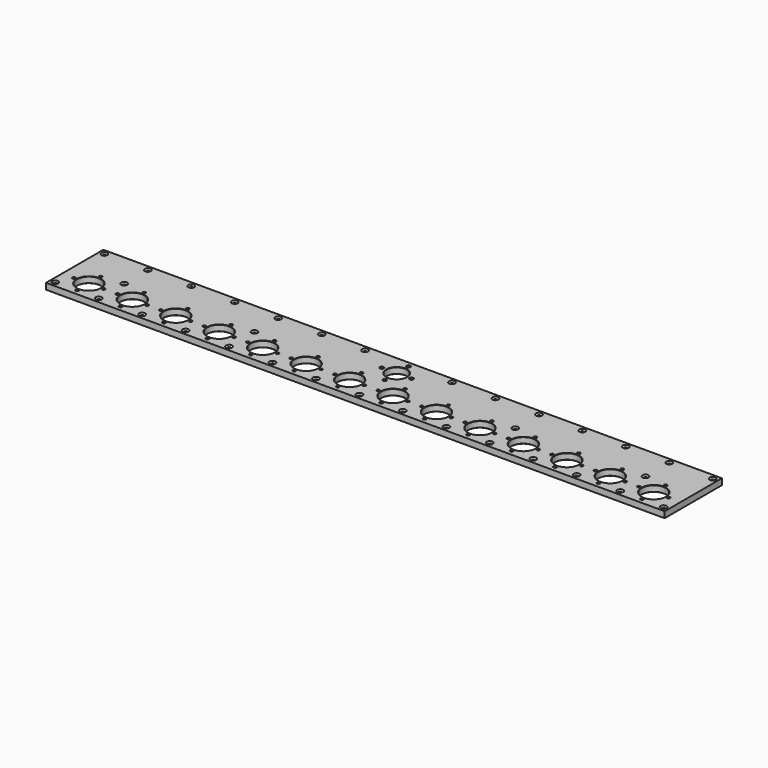
from build123d import *

# Parameters (mm, degrees)
F0_W     = 1210
F0_H     = 140
F0_R     = 3.25
F0_R_2   = 2.5
F0_R_3   = 23.5
F0_R_4   = 20
F1_DEPTH = 12
F2_SIZE  = 0.5
F4_SIZE  = 2.75


# Not quite as in the source:
# - two fillets or chamfers of one size are made in one step
# - a feature of the source that left no trace in its solid (it failed there, or was rolled back) is left out


with BuildPart() as f1:
    # F0 (on Top) → F1 (new body)
    with BuildSketch(Plane.XY):
        with Locations((0, -31)):
            Rectangle(F0_W, F0_H)
        with Locations((-595, -91)):
            Circle(F0_R, mode=Mode.SUBTRACT)
        with Locations((-552.5, -91)):
            Circle(F0_R_2, mode=Mode.SUBTRACT)
        with Locations((-510, -91)):
            Circle(F0_R, mode=Mode.SUBTRACT)
        with Locations((-467.5, -91)):
            Circle(F0_R_2, mode=Mode.SUBTRACT)
        with Locations((-425, -91)):
            Circle(F0_R, mode=Mode.SUBTRACT)
        with Locations((-382.5, -91)):
            Circle(F0_R_2, mode=Mode.SUBTRACT)
        with Locations((-340, -91)):
            Circle(F0_R, mode=Mode.SUBTRACT)
        with Locations((-297.5, -91)):
            Circle(F0_R_2, mode=Mode.SUBTRACT)
        with Locations((-255, -91)):
            Circle(F0_R, mode=Mode.SUBTRACT)
        with Locations((-212.5, -91)):
            Circle(F0_R_2, mode=Mode.SUBTRACT)
        with Locations((-170, -91)):
            Circle(F0_R, mode=Mode.SUBTRACT)
        with Locations((-127.5, -91)):
            Circle(F0_R_2, mode=Mode.SUBTRACT)
        with Locations((-85, -91)):
            Circle(F0_R, mode=Mode.SUBTRACT)
        with Locations((-42.5, -91)):
            Circle(F0_R_2, mode=Mode.SUBTRACT)
        with Locations((-581.5, -62)):
            Circle(F0_R_2, mode=Mode.SUBTRACT)
        with Locations((-552.5, -62)):
            Circle(F0_R_3, mode=Mode.SUBTRACT)
        with Locations((-523.5, -62)):
            Circle(F0_R_2, mode=Mode.SUBTRACT)
        with Locations((-496.5, -62)):
            Circle(F0_R_2, mode=Mode.SUBTRACT)
        with Locations((-467.5, -62)):
            Circle(F0_R_3, mode=Mode.SUBTRACT)
        with Locations((-438.5, -62)):
            Circle(F0_R_2, mode=Mode.SUBTRACT)
        with Locations((-411.5, -62)):
            Circle(F0_R_2, mode=Mode.SUBTRACT)
        with Locations((-382.5, -62)):
            Circle(F0_R_3, mode=Mode.SUBTRACT)
        with Locations((-353.5, -62)):
            Circle(F0_R_2, mode=Mode.SUBTRACT)
        with Locations((-326.5, -62)):
            Circle(F0_R_2, mode=Mode.SUBTRACT)
        with Locations((-552.5, -33)):
            Circle(F0_R_2, mode=Mode.SUBTRACT)
        with Locations((-467.5, -33)):
            Circle(F0_R_2, mode=Mode.SUBTRACT)
        with Locations((-382.5, -33)):
            Circle(F0_R_2, mode=Mode.SUBTRACT)
        with Locations((-297.5, -62)):
            Circle(F0_R_3, mode=Mode.SUBTRACT)
        with Locations((-268.5, -62)):
            Circle(F0_R_2, mode=Mode.SUBTRACT)
        with Locations((-241.5, -62)):
            Circle(F0_R_2, mode=Mode.SUBTRACT)
        with Locations((-212.5, -62)):
            Circle(F0_R_3, mode=Mode.SUBTRACT)
        with Locations((-183.5, -62)):
            Circle(F0_R_2, mode=Mode.SUBTRACT)
        with Locations((-156.5, -62)):
            Circle(F0_R_2, mode=Mode.SUBTRACT)
        with Locations((-127.5, -62)):
            Circle(F0_R_3, mode=Mode.SUBTRACT)
        with Locations((-98.5, -62)):
            Circle(F0_R_2, mode=Mode.SUBTRACT)
        with Locations((-71.5, -62)):
            Circle(F0_R_2, mode=Mode.SUBTRACT)
        with Locations((-42.5, -62)):
            Circle(F0_R_3, mode=Mode.SUBTRACT)
        with Locations((-13.5, -62)):
            Circle(F0_R_2, mode=Mode.SUBTRACT)
        with Locations((-297.5, -33)):
            Circle(F0_R_2, mode=Mode.SUBTRACT)
        with Locations((-212.5, -33)):
            Circle(F0_R_2, mode=Mode.SUBTRACT)
        with Locations((-127.5, -33)):
            Circle(F0_R_2, mode=Mode.SUBTRACT)
        with Locations((-42.5, -33)):
            Circle(F0_R_2, mode=Mode.SUBTRACT)
        with Locations((0, -91)):
            Circle(F0_R, mode=Mode.SUBTRACT)
        with Locations((42.5, -91)):
            Circle(F0_R_2, mode=Mode.SUBTRACT)
        with Locations((85, -91)):
            Circle(F0_R, mode=Mode.SUBTRACT)
        with Locations((127.5, -91)):
            Circle(F0_R_2, mode=Mode.SUBTRACT)
        with Locations((170, -91)):
            Circle(F0_R, mode=Mode.SUBTRACT)
        with Locations((212.5, -91)):
            Circle(F0_R_2, mode=Mode.SUBTRACT)
        with Locations((255, -91)):
            Circle(F0_R, mode=Mode.SUBTRACT)
        with Locations((297.5, -91)):
            Circle(F0_R_2, mode=Mode.SUBTRACT)
        with Locations((340, -91)):
            Circle(F0_R, mode=Mode.SUBTRACT)
        with Locations((382.5, -91)):
            Circle(F0_R_2, mode=Mode.SUBTRACT)
        with Locations((425, -91)):
            Circle(F0_R, mode=Mode.SUBTRACT)
        with Locations((467.5, -91)):
            Circle(F0_R_2, mode=Mode.SUBTRACT)
        with Locations((510, -91)):
            Circle(F0_R, mode=Mode.SUBTRACT)
        with Locations((552.5, -91)):
            Circle(F0_R_2, mode=Mode.SUBTRACT)
        with Locations((595, -91)):
            Circle(F0_R, mode=Mode.SUBTRACT)
        with Locations((13.5, -62)):
            Circle(F0_R_2, mode=Mode.SUBTRACT)
        with Locations((42.5, -62)):
            Circle(F0_R_3, mode=Mode.SUBTRACT)
        with Locations((71.5, -62)):
            Circle(F0_R_2, mode=Mode.SUBTRACT)
        with Locations((98.5, -62)):
            Circle(F0_R_2, mode=Mode.SUBTRACT)
        with Locations((127.5, -62)):
            Circle(F0_R_3, mode=Mode.SUBTRACT)
        with Locations((156.5, -62)):
            Circle(F0_R_2, mode=Mode.SUBTRACT)
        with Locations((183.5, -62)):
            Circle(F0_R_2, mode=Mode.SUBTRACT)
        with Locations((212.5, -62)):
            Circle(F0_R_3, mode=Mode.SUBTRACT)
        with Locations((241.5, -62)):
            Circle(F0_R_2, mode=Mode.SUBTRACT)
        with Locations((268.5, -62)):
            Circle(F0_R_2, mode=Mode.SUBTRACT)
        with Locations((297.5, -62)):
            Circle(F0_R_3, mode=Mode.SUBTRACT)
        with Locations((42.5, -33)):
            Circle(F0_R_2, mode=Mode.SUBTRACT)
        with Locations((127.5, -33)):
            Circle(F0_R_2, mode=Mode.SUBTRACT)
        with Locations((212.5, -33)):
            Circle(F0_R_2, mode=Mode.SUBTRACT)
        with Locations((297.5, -33)):
            Circle(F0_R_2, mode=Mode.SUBTRACT)
        with Locations((326.5, -62)):
            Circle(F0_R_2, mode=Mode.SUBTRACT)
        with Locations((353.5, -62)):
            Circle(F0_R_2, mode=Mode.SUBTRACT)
        with Locations((382.5, -62)):
            Circle(F0_R_3, mode=Mode.SUBTRACT)
        with Locations((411.5, -62)):
            Circle(F0_R_2, mode=Mode.SUBTRACT)
        with Locations((438.5, -62)):
            Circle(F0_R_2, mode=Mode.SUBTRACT)
        with Locations((467.5, -62)):
            Circle(F0_R_3, mode=Mode.SUBTRACT)
        with Locations((496.5, -62)):
            Circle(F0_R_2, mode=Mode.SUBTRACT)
        with Locations((523.5, -62)):
            Circle(F0_R_2, mode=Mode.SUBTRACT)
        with Locations((552.5, -62)):
            Circle(F0_R_3, mode=Mode.SUBTRACT)
        with Locations((581.5, -62)):
            Circle(F0_R_2, mode=Mode.SUBTRACT)
        with Locations((382.5, -33)):
            Circle(F0_R_2, mode=Mode.SUBTRACT)
        with Locations((467.5, -33)):
            Circle(F0_R_2, mode=Mode.SUBTRACT)
        with Locations((552.5, -33)):
            Circle(F0_R_2, mode=Mode.SUBTRACT)
        with Locations((-510, -29)):
            Circle(F0_R, mode=Mode.SUBTRACT)
        with Locations((-255, -29)):
            Circle(F0_R, mode=Mode.SUBTRACT)
        with Locations((-29, 0)):
            Circle(F0_R, mode=Mode.SUBTRACT)
        with Locations((-595, 29)):
            Circle(F0_R, mode=Mode.SUBTRACT)
        with Locations((-510, 29)):
            Circle(F0_R, mode=Mode.SUBTRACT)
        with Locations((-425, 29)):
            Circle(F0_R, mode=Mode.SUBTRACT)
        with Locations((-340, 29)):
            Circle(F0_R, mode=Mode.SUBTRACT)
        with Locations((-255, 29)):
            Circle(F0_R, mode=Mode.SUBTRACT)
        with Locations((-170, 29)):
            Circle(F0_R, mode=Mode.SUBTRACT)
        with Locations((-85, 29)):
            Circle(F0_R, mode=Mode.SUBTRACT)
        with Locations((0, -29)):
            Circle(F0_R, mode=Mode.SUBTRACT)
        with Locations((255, -29)):
            Circle(F0_R, mode=Mode.SUBTRACT)
        Circle(F0_R_4, mode=Mode.SUBTRACT)
        with Locations((29, 0)):
            Circle(F0_R, mode=Mode.SUBTRACT)
        with Locations((510, -29)):
            Circle(F0_R, mode=Mode.SUBTRACT)
        with Locations((0, 29)):
            Circle(F0_R, mode=Mode.SUBTRACT)
        with Locations((85, 29)):
            Circle(F0_R, mode=Mode.SUBTRACT)
        with Locations((170, 29)):
            Circle(F0_R, mode=Mode.SUBTRACT)
        with Locations((255, 29)):
            Circle(F0_R, mode=Mode.SUBTRACT)
        with Locations((340, 29)):
            Circle(F0_R, mode=Mode.SUBTRACT)
        with Locations((425, 29)):
            Circle(F0_R, mode=Mode.SUBTRACT)
        with Locations((510, 29)):
            Circle(F0_R, mode=Mode.SUBTRACT)
        with Locations((595, 29)):
            Circle(F0_R, mode=Mode.SUBTRACT)
    extrude(amount=F1_DEPTH)

    # F2
    f2_edges = [f1.edges().sort_by_distance(p)[0] for p in [
        (576, -62, 6),
        (529, -62, 0),
        (529, -62, 12),
        (526, -62, 6),
        (521, -62, 0),
        (521, -62, 12),
        (555, -91, 6),
        (550, -91, 0),
        (550, -91, 12),
        (555, -33, 6),
        (550, -33, 0),
        (550, -33, 12),
        (584, -62, 6),
        (579, -62, 0),
        (579, -62, 12),
        (491, -62, 6),
        (444, -62, 0),
        (444, -62, 12),
        (406, -62, 6),
        (359, -62, 0),
        (359, -62, 12),
        (321, -62, 6),
        (274, -62, 0),
        (274, -62, 12),
        (236, -62, 6),
        (189, -62, 0),
        (189, -62, 12),
        (151, -62, 6),
        (104, -62, 0),
        (104, -62, 12),
        (66, -62, 6),
        (19, -62, 0),
        (19, -62, 12),
        (-19, -62, 6),
        (-66, -62, 0),
        (-66, -62, 12),
        (-104, -62, 6),
        (-151, -62, 0),
        (-151, -62, 12),
        (-189, -62, 6),
        (-236, -62, 0),
        (-236, -62, 12),
        (-274, -62, 6),
        (-321, -62, 0),
        (-321, -62, 12),
        (-359, -62, 6),
        (-406, -62, 0),
        (-406, -62, 12),
        (-444, -62, 6),
        (-491, -62, 0),
        (-491, -62, 12),
        (-529, -62, 6),
        (-576, -62, 0),
        (-576, -62, 12),
        (-579, -62, 6),
        (-584, -62, 0),
        (-584, -62, 12),
        (-550, -91, 6),
        (-555, -91, 0),
        (-555, -91, 12),
        (-521, -62, 6),
        (-526, -62, 0),
        (-526, -62, 12),
        (-550, -33, 6),
        (-555, -33, 0),
        (-555, -33, 12),
        (20, 0, 6),
        (-20, 0, 0),
        (-20, 0, 12),
        (-598.25, -91, 0),
        (-513.25, -91, 0),
        (-470, -91, 0),
        (-470, -91, 12),
        (-428.25, -91, 0),
        (-385, -91, 0),
        (-385, -91, 12),
        (-343.25, -91, 0),
        (-300, -91, 0),
        (-300, -91, 12),
        (-258.25, -91, 0),
        (-215, -91, 0),
        (-215, -91, 12),
        (-173.25, -91, 0),
        (-130, -91, 0),
        (-130, -91, 12),
        (-88.25, -91, 0),
        (-45, -91, 0),
        (-45, -91, 12),
        (-499, -62, 0),
        (-499, -62, 12),
        (-441, -62, 0),
        (-441, -62, 12),
        (-414, -62, 0),
        (-414, -62, 12),
        (-356, -62, 0),
        (-356, -62, 12),
        (-329, -62, 0),
        (-329, -62, 12),
        (-470, -33, 0),
        (-470, -33, 12),
        (-385, -33, 0),
        (-385, -33, 12),
        (-271, -62, 0),
        (-271, -62, 12),
        (-244, -62, 0),
        (-244, -62, 12),
        (-186, -62, 0),
        (-186, -62, 12),
        (-159, -62, 0),
        (-159, -62, 12),
        (-101, -62, 0),
        (-101, -62, 12),
        (-74, -62, 0),
        (-74, -62, 12),
        (-16, -62, 0),
        (-16, -62, 12),
        (-300, -33, 0),
        (-300, -33, 12),
        (-215, -33, 0),
        (-215, -33, 12),
        (-130, -33, 0),
        (-130, -33, 12),
        (-45, -33, 0),
        (-45, -33, 12),
        (-3.25, -91, 0),
        (40, -91, 0),
        (40, -91, 12),
        (81.75, -91, 0),
        (125, -91, 0),
        (125, -91, 12),
        (166.75, -91, 0),
        (210, -91, 0),
        (210, -91, 12),
        (251.75, -91, 0),
        (295, -91, 0),
        (295, -91, 12),
        (336.75, -91, 0),
        (380, -91, 0),
        (380, -91, 12),
        (421.75, -91, 0),
        (465, -91, 0),
        (465, -91, 12),
        (506.75, -91, 0),
        (591.75, -91, 0),
        (11, -62, 0),
        (11, -62, 12),
        (69, -62, 0),
        (69, -62, 12),
        (96, -62, 0),
        (96, -62, 12),
        (154, -62, 0),
        (154, -62, 12),
        (181, -62, 0),
        (181, -62, 12),
        (239, -62, 0),
        (239, -62, 12),
        (266, -62, 0),
        (266, -62, 12),
        (40, -33, 0),
        (40, -33, 12),
        (125, -33, 0),
        (210, -33, 0),
        (210, -33, 12),
        (295, -33, 0),
        (295, -33, 12),
        (324, -62, 0),
        (324, -62, 12),
        (351, -62, 0),
        (351, -62, 12),
        (409, -62, 0),
        (409, -62, 12),
        (436, -62, 0),
        (436, -62, 12),
        (494, -62, 0),
        (494, -62, 12),
        (380, -33, 0),
        (380, -33, 12),
        (465, -33, 0),
        (465, -33, 12),
        (-513.25, -29, 0),
        (-258.25, -29, 0),
        (-32.25, 0, 0),
        (-32.25, 0, 12),
        (-598.25, 29, 0),
        (-513.25, 29, 0),
        (-428.25, 29, 0),
        (-343.25, 29, 0),
        (-258.25, 29, 0),
        (-173.25, 29, 0),
        (-88.25, 29, 0),
        (-3.25, -29, 0),
        (-3.25, -29, 12),
        (251.75, -29, 0),
        (25.75, 0, 0),
        (25.75, 0, 12),
        (506.75, -29, 0),
        (-3.25, 29, 0),
        (-3.25, 29, 12),
        (81.75, 29, 0),
        (166.75, 29, 0),
        (251.75, 29, 0),
        (336.75, 29, 0),
        (421.75, 29, 0),
        (506.75, 29, 0),
        (591.75, 29, 0),
    ]]
    chamfer(f2_edges, length=F2_SIZE)

    # F4
    f4_edges = [f1.edges().sort_by_distance(p)[0] for p in [
        (-598.25, 29, 12),
        (-598.25, -91, 12),
        (-513.25, -29, 12),
        (-513.25, 29, 12),
        (-513.25, -91, 12),
        (-428.25, -91, 12),
        (-428.25, 29, 12),
        (-343.25, -91, 12),
        (-343.25, 29, 12),
        (-258.25, -91, 12),
        (-258.25, 29, 12),
        (-258.25, -29, 12),
        (-173.25, 29, 12),
        (-173.25, -91, 12),
        (-88.25, 29, 12),
        (-3.25, -91, 12),
        (-88.25, -91, 12),
        (81.75, -91, 12),
        (81.75, 29, 12),
        (166.75, 29, 12),
        (166.75, -91, 12),
        (251.75, -91, 12),
        (251.75, -29, 12),
        (251.75, 29, 12),
        (336.75, -91, 12),
        (336.75, 29, 12),
        (421.75, 29, 12),
        (506.75, -91, 12),
        (506.75, 29, 12),
        (421.75, -91, 12),
        (591.75, -91, 12),
        (591.75, 29, 12),
        (506.75, -29, 12),
    ]]
    chamfer(f4_edges, length=F4_SIZE)


solid = f1.part
